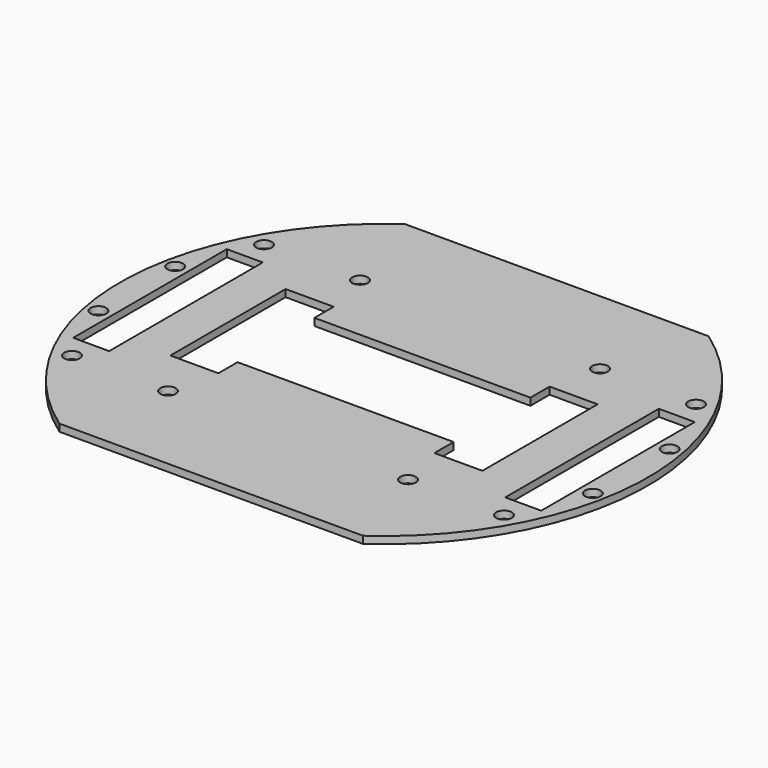
from build123d import *

# Parameters (mm, degrees)
F1_DEPTH = 3
F3_D     = 6.5
F5_D     = 6.5
F6_W     = 90
F6_H     = 40
F7_DEPTH = 3.001
F9_DEPTH = 3.001


# Not quite as in the source:
# - a feature names something its author has since deleted; it is built from what else it names


with BuildPart() as f1:
    # F0 (on Top) → F1 (new body)
    with BuildSketch(Plane.XY):
        with BuildLine():
            Line((63.2455532034, 90), (-63.2455532034, 90))
            ThreePointArc((-63.2455532034, 90), (-110, 0), (-63.2455532034, -90))
            Line((-63.2455532034, -90), (63.2455532034, -90))
            ThreePointArc((63.2455532034, -90), (110, 0), (63.2455532034, 90))
        make_face()
    extrude(amount=F1_DEPTH)

    # F3 (through all)
    with Locations(Plane.XY.offset(3)):
        with Locations((-103, 20), (-103, -20), (-90, 50), (-90, -50), (90, -50), (90, 50), (103, 20), (103, -20)):
            Hole(F3_D / 2)

    # F5 (through all)
    with Locations(Plane.XY.offset(3)):
        with Locations((-50, 50), (50, 50), (50, -50), (-50, -50)):
            Hole(F5_D / 2)

    # F6 (on face) → F7 (cut, through all)
    with BuildSketch(Plane.XY.offset(3)):
        Polygon((-45, -20), (-45, 20), (-45, 30), (-65, 30), (-65, -30), (-45, -30), align=None)
        Rectangle(F6_W, F6_H)
        Polygon((45, 30), (45, 20), (45, -20), (45, -30), (65, -30), (65, 30), align=None)
    extrude(amount=-F7_DEPTH, mode=Mode.SUBTRACT)

    # F8 (on face) → F9 (cut, through all)
    with BuildSketch(Plane.XY.offset(3)):
        Polygon((-90, 40), (-97.5, 40), (-97.5, -40), (-82.5, -40), (-82.5, 40), align=None)
        Polygon((90, 40), (82.5, 40), (82.5, -40), (97.5, -40), (97.5, 40), align=None)
    extrude(amount=-F9_DEPTH, mode=Mode.SUBTRACT)


solid = f1.part
